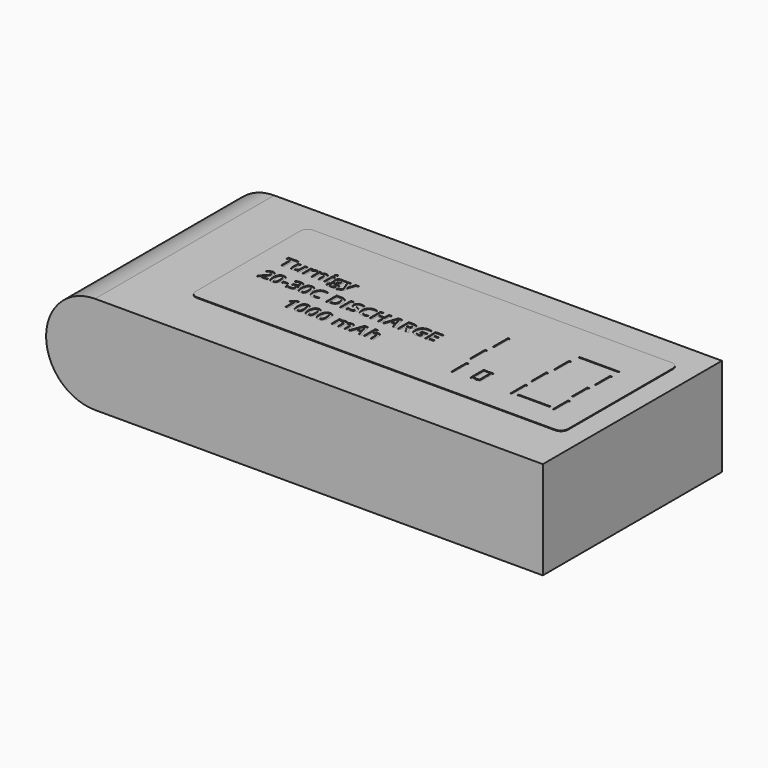
from build123d import *

# Parameters (mm, degrees)
F0_W     = 71
F0_H     = 32
F1_DEPTH = 14
F2_R     = 6.99999
F3_W     = 0.296875
F3_H     = 2.7330729167
F3_W_2   = 0.7282986111
F3_H_2   = 0.3389756944
F3_W_3   = 0.4205729167
F3_H_3   = 1.9830729167
F3_W_4   = 0.4136284722
F3_H_4   = 1.5164930556
F4_DEPTH = 0.1


# Not quite as in the source:
# - a fillet or chamfer is up to 0.001 mm smaller than in the source, because OpenCascade refuses the exact size


with BuildPart() as f1:
    # F0 (on Top) → F1 (new body)
    with BuildSketch(Plane.XY):
        with Locations((-5.0565935671, -0.0620016182)):
            Rectangle(F0_W, F0_H)
    extrude(amount=F1_DEPTH)

    # F2 (radius 7 in the source; OpenCascade refuses exactly that, so slightly less here)
    f2_edges = [f1.edges().sort_by_distance(p)[0] for p in [
        (-40.556594, -0.062002, 14),
        (-40.556594, -0.062002, 0),
    ]]
    fillet(f2_edges, radius=F2_R)

    # F3 (on face) → F4 (join)
    with BuildSketch(Plane.XY.offset(14)):
        with BuildLine():
            Line((26.4446923286, 11.9373770431), (-24.7810670882, 11.9373770431))
            ThreePointArc((-24.7810670882, 11.9373770431), (-25.4881738694, 11.6444838243), (-25.7810670882, 10.9373770431))
            Line((-25.7810670882, 10.9373770431), (-25.7810670882, -7.8157188147))
            ThreePointArc((-25.7810670882, -7.8157188147), (-25.4881738694, -8.5228255959), (-24.7810670882, -8.8157188147))
            Line((-24.7810670882, -8.8157188147), (26.4446923286, -8.8157188147))
            ThreePointArc((26.4446923286, -8.8157188147), (27.1517991098, -8.5228255959), (27.4446923286, -7.8157188147))
            Line((27.4446923286, -7.8157188147), (27.4446923286, 10.9373770431))
            ThreePointArc((27.4446923286, 10.9373770431), (27.1517991098, 11.6444838243), (26.4446923286, 11.9373770431))
        make_face()
        with BuildLine():
            Line((-15.2074745615, -2.5303943503), (-15.2074745615, -4.5134672669))
            Line((-15.2074745615, -4.5134672669), (-15.6267453948, -4.5134672669))
            Line((-15.6267453948, -4.5134672669), (-15.6267453948, -3.3658978225))
            Line((-15.6267453948, -3.3658978225), (-15.6224051171, -3.1775297669))
            Line((-15.6224051171, -3.1775297669), (-15.6158947004, -2.9713665725))
            add(Edge.make_bspline(
                [(-15.6158947004, -2.9713665725), (-15.7200613671, -3.0755332392), (-15.7608599782, -3.1080853225)],
                knots=[0, 0, 0, 1, 1, 1], degree=2))
            Line((-15.7608599782, -3.1080853225), (-15.9887245615, -3.2912450447))
            Line((-15.9887245615, -3.2912450447), (-16.190981506, -3.0390749058))
            Line((-16.190981506, -3.0390749058), (-15.5520926171, -2.5303943503))
            Line((-15.5520926171, -2.5303943503), (-15.2074745615, -2.5303943503))
        make_face(mode=Mode.SUBTRACT)
        with BuildLine():
            add(Edge.make_bspline(
                [(-13.458559631, -2.7595610169), (-13.2829953948, -3.0199776836), (-13.2829953948, -3.5221478225)],
                knots=[0, 0, 0, 1, 1, 1], degree=2))
            add(Edge.make_bspline(
                [(-13.2829953948, -3.5221478225), (-13.2829953948, -4.0412450447), (-13.4531342837, -4.2910280308)],
                knots=[0, 0, 0, 1, 1, 1], degree=2))
            add(Edge.make_bspline(
                [(-13.4531342837, -4.2910280308), (-13.6232731726, -4.5408110169), (-13.9774398393, -4.5408110169)],
                knots=[0, 0, 0, 1, 1, 1], degree=2))
            add(Edge.make_bspline(
                [(-13.9774398393, -4.5408110169), (-14.3207558115, -4.5408110169), (-14.4950179643, -4.2829985169)],
                knots=[0, 0, 0, 1, 1, 1], degree=2))
            add(Edge.make_bspline(
                [(-14.4950179643, -4.2829985169), (-14.6692801171, -4.0251860169), (-14.6692801171, -3.5221478225)],
                knots=[0, 0, 0, 1, 1, 1], degree=2))
            add(Edge.make_bspline(
                [(-14.6692801171, -3.5221478225), (-14.6692801171, -2.9969742114), (-14.499575256, -2.7480592808)],
                knots=[0, 0, 0, 1, 1, 1], degree=2))
            add(Edge.make_bspline(
                [(-14.499575256, -2.7480592808), (-14.3298703948, -2.4991443503), (-13.9774398393, -2.4991443503)],
                knots=[0, 0, 0, 1, 1, 1], degree=2))
            add(Edge.make_bspline(
                [(-13.9774398393, -2.4991443503), (-13.6341238671, -2.4991443503), (-13.458559631, -2.7595610169)],
                knots=[0, 0, 0, 1, 1, 1], degree=2))
        make_face(mode=Mode.SUBTRACT)
        with BuildLine():
            add(Edge.make_bspline(
                [(-11.8730561587, -2.7595610169), (-11.6974919226, -3.0199776836), (-11.6974919226, -3.5221478225)],
                knots=[0, 0, 0, 1, 1, 1], degree=2))
            add(Edge.make_bspline(
                [(-11.6974919226, -3.5221478225), (-11.6974919226, -4.0412450447), (-11.8676308115, -4.2910280308)],
                knots=[0, 0, 0, 1, 1, 1], degree=2))
            add(Edge.make_bspline(
                [(-11.8676308115, -4.2910280308), (-12.0377697004, -4.5408110169), (-12.3919363671, -4.5408110169)],
                knots=[0, 0, 0, 1, 1, 1], degree=2))
            add(Edge.make_bspline(
                [(-12.3919363671, -4.5408110169), (-12.7352523393, -4.5408110169), (-12.9095144921, -4.2829985169)],
                knots=[0, 0, 0, 1, 1, 1], degree=2))
            add(Edge.make_bspline(
                [(-12.9095144921, -4.2829985169), (-13.0837766448, -4.0251860169), (-13.0837766448, -3.5221478225)],
                knots=[0, 0, 0, 1, 1, 1], degree=2))
            add(Edge.make_bspline(
                [(-13.0837766448, -3.5221478225), (-13.0837766448, -2.9969742114), (-12.9140717837, -2.7480592808)],
                knots=[0, 0, 0, 1, 1, 1], degree=2))
            add(Edge.make_bspline(
                [(-12.9140717837, -2.7480592808), (-12.7443669226, -2.4991443503), (-12.3919363671, -2.4991443503)],
                knots=[0, 0, 0, 1, 1, 1], degree=2))
            add(Edge.make_bspline(
                [(-12.3919363671, -2.4991443503), (-12.0486203948, -2.4991443503), (-11.8730561587, -2.7595610169)],
                knots=[0, 0, 0, 1, 1, 1], degree=2))
        make_face(mode=Mode.SUBTRACT)
        with BuildLine():
            add(Edge.make_bspline(
                [(-10.2875526865, -2.7595610169), (-10.1119884504, -3.0199776836), (-10.1119884504, -3.5221478225)],
                knots=[0, 0, 0, 1, 1, 1], degree=2))
            add(Edge.make_bspline(
                [(-10.1119884504, -3.5221478225), (-10.1119884504, -4.0412450447), (-10.2821273393, -4.2910280308)],
                knots=[0, 0, 0, 1, 1, 1], degree=2))
            add(Edge.make_bspline(
                [(-10.2821273393, -4.2910280308), (-10.4522662282, -4.5408110169), (-10.8064328948, -4.5408110169)],
                knots=[0, 0, 0, 1, 1, 1], degree=2))
            add(Edge.make_bspline(
                [(-10.8064328948, -4.5408110169), (-11.1497488671, -4.5408110169), (-11.3240110198, -4.2829985169)],
                knots=[0, 0, 0, 1, 1, 1], degree=2))
            add(Edge.make_bspline(
                [(-11.3240110198, -4.2829985169), (-11.4982731726, -4.0251860169), (-11.4982731726, -3.5221478225)],
                knots=[0, 0, 0, 1, 1, 1], degree=2))
            add(Edge.make_bspline(
                [(-11.4982731726, -3.5221478225), (-11.4982731726, -2.9969742114), (-11.3285683115, -2.7480592808)],
                knots=[0, 0, 0, 1, 1, 1], degree=2))
            add(Edge.make_bspline(
                [(-11.3285683115, -2.7480592808), (-11.1588634504, -2.4991443503), (-10.8064328948, -2.4991443503)],
                knots=[0, 0, 0, 1, 1, 1], degree=2))
            add(Edge.make_bspline(
                [(-10.8064328948, -2.4991443503), (-10.4631169226, -2.4991443503), (-10.2875526865, -2.7595610169)],
                knots=[0, 0, 0, 1, 1, 1], degree=2))
        make_face(mode=Mode.SUBTRACT)
        with BuildLine():
            Line((-7.7165891448, -3.7526165725), (-7.7165891448, -4.5134672669))
            Line((-7.7165891448, -4.5134672669), (-8.1302176171, -4.5134672669))
            Line((-8.1302176171, -4.5134672669), (-8.1302176171, -3.6276165725))
            add(Edge.make_bspline(
                [(-8.1302176171, -3.6276165725), (-8.1302176171, -3.4635540725), (-8.185122131, -3.3815228225)],
                knots=[0, 0, 0, 1, 1, 1], degree=2))
            add(Edge.make_bspline(
                [(-8.185122131, -3.3815228225), (-8.2400266448, -3.2994915725), (-8.3580822004, -3.2994915725)],
                knots=[0, 0, 0, 1, 1, 1], degree=2))
            add(Edge.make_bspline(
                [(-8.3580822004, -3.2994915725), (-8.5169363671, -3.2994915725), (-8.5887679643, -3.4162450447)],
                knots=[0, 0, 0, 1, 1, 1], degree=2))
            add(Edge.make_bspline(
                [(-8.5887679643, -3.4162450447), (-8.6605995615, -3.5329985169), (-8.6605995615, -3.7999256003)],
                knots=[0, 0, 0, 1, 1, 1], degree=2))
            Line((-8.6605995615, -3.7999256003), (-8.6605995615, -4.5134672669))
            Line((-8.6605995615, -4.5134672669), (-9.0742280337, -4.5134672669))
            Line((-9.0742280337, -4.5134672669), (-9.0742280337, -2.9969742114))
            Line((-9.0742280337, -2.9969742114), (-8.7582558115, -2.9969742114))
            Line((-8.7582558115, -2.9969742114), (-8.702700256, -3.1909846281))
            Line((-8.702700256, -3.1909846281), (-8.6796967837, -3.1909846281))
            add(Edge.make_bspline(
                [(-8.6796967837, -3.1909846281), (-8.6184988671, -3.0863839336), (-8.5032644921, -3.0275731697)],
                knots=[0, 0, 0, 1, 1, 1], degree=2))
            add(Edge.make_bspline(
                [(-8.5032644921, -3.0275731697), (-8.3880301171, -2.9687624058), (-8.2387245615, -2.9687624058)],
                knots=[0, 0, 0, 1, 1, 1], degree=2))
            add(Edge.make_bspline(
                [(-8.2387245615, -2.9687624058), (-7.8984467837, -2.9687624058), (-7.7773530337, -3.1909846281)],
                knots=[0, 0, 0, 1, 1, 1], degree=2))
            Line((-7.7773530337, -3.1909846281), (-7.7408947004, -3.1909846281))
            add(Edge.make_bspline(
                [(-7.7408947004, -3.1909846281), (-7.6796967837, -3.0850818503), (-7.5612072004, -3.0269221281)],
                knots=[0, 0, 0, 1, 1, 1], degree=2))
            add(Edge.make_bspline(
                [(-7.5612072004, -3.0269221281), (-7.4427176171, -2.9687624058), (-7.2934120615, -2.9687624058)],
                knots=[0, 0, 0, 1, 1, 1], degree=2))
            add(Edge.make_bspline(
                [(-7.2934120615, -2.9687624058), (-7.0355995615, -2.9687624058), (-6.9034381032, -3.1009238642)],
                knots=[0, 0, 0, 1, 1, 1], degree=2))
            add(Edge.make_bspline(
                [(-6.9034381032, -3.1009238642), (-6.7712766448, -3.2330853225), (-6.7712766448, -3.5247519892)],
                knots=[0, 0, 0, 1, 1, 1], degree=2))
            Line((-6.7712766448, -3.5247519892), (-6.7712766448, -4.5134672669))
            Line((-6.7712766448, -4.5134672669), (-7.1862072004, -4.5134672669))
            Line((-7.1862072004, -4.5134672669), (-7.1862072004, -3.6276165725))
            add(Edge.make_bspline(
                [(-7.1862072004, -3.6276165725), (-7.1862072004, -3.4635540725), (-7.2411117143, -3.3815228225)],
                knots=[0, 0, 0, 1, 1, 1], degree=2))
            add(Edge.make_bspline(
                [(-7.2411117143, -3.3815228225), (-7.2960162282, -3.2994915725), (-7.4140717837, -3.2994915725)],
                knots=[0, 0, 0, 1, 1, 1], degree=2))
            add(Edge.make_bspline(
                [(-7.4140717837, -3.2994915725), (-7.565981506, -3.2994915725), (-7.6412853254, -3.4079985169)],
                knots=[0, 0, 0, 1, 1, 1], degree=2))
            add(Edge.make_bspline(
                [(-7.6412853254, -3.4079985169), (-7.7165891448, -3.5165054614), (-7.7165891448, -3.7526165725)],
                knots=[0, 0, 0, 1, 1, 1], degree=2))
        make_face(mode=Mode.SUBTRACT)
        Polygon((-4.6471447004, -4.5134672669), (-5.1002697004, -4.5134672669), (-5.2439328948, -4.0412450447), (-5.9670231726, -4.0412450447), (-6.1106863671, -4.5134672669), (-6.5638113671, -4.5134672669), (-5.8637245615, -2.5221478225), (-5.3498356726, -2.5221478225), align=None, mode=Mode.SUBTRACT)
        with BuildLine():
            Line((-3.0303912282, -3.5247519892), (-3.0303912282, -4.5134672669))
            Line((-3.0303912282, -4.5134672669), (-3.4440197004, -4.5134672669))
            Line((-3.4440197004, -4.5134672669), (-3.4440197004, -3.6276165725))
            add(Edge.make_bspline(
                [(-3.4440197004, -3.6276165725), (-3.4440197004, -3.2994915725), (-3.6883773393, -3.2994915725)],
                knots=[0, 0, 0, 1, 1, 1], degree=2))
            add(Edge.make_bspline(
                [(-3.6883773393, -3.2994915725), (-3.8619884504, -3.2994915725), (-3.9392453948, -3.4175471281)],
                knots=[0, 0, 0, 1, 1, 1], degree=2))
            add(Edge.make_bspline(
                [(-3.9392453948, -3.4175471281), (-4.0165023393, -3.5356026836), (-4.0165023393, -3.7999256003)],
                knots=[0, 0, 0, 1, 1, 1], degree=2))
            Line((-4.0165023393, -3.7999256003), (-4.0165023393, -4.5134672669))
            Line((-4.0165023393, -4.5134672669), (-4.4301308115, -4.5134672669))
            Line((-4.4301308115, -4.5134672669), (-4.4301308115, -2.4027901836))
            Line((-4.4301308115, -2.4027901836), (-4.0165023393, -2.4027901836))
            Line((-4.0165023393, -2.4027901836), (-4.0165023393, -2.8329117114))
            add(Edge.make_bspline(
                [(-4.0165023393, -2.8329117114), (-4.0165023393, -2.8832589336), (-4.0260509504, -3.0690228225)],
                knots=[0, 0, 0, 1, 1, 1], degree=2))
            Line((-4.0260509504, -3.0690228225), (-4.0355995615, -3.1909846281))
            Line((-4.0355995615, -3.1909846281), (-4.0138981726, -3.1909846281))
            add(Edge.make_bspline(
                [(-4.0138981726, -3.1909846281), (-3.8754433115, -2.9687624058), (-3.5742280337, -2.9687624058)],
                knots=[0, 0, 0, 1, 1, 1], degree=2))
            add(Edge.make_bspline(
                [(-3.5742280337, -2.9687624058), (-3.3068669226, -2.9687624058), (-3.1686290754, -3.1124256003)],
                knots=[0, 0, 0, 1, 1, 1], degree=2))
            add(Edge.make_bspline(
                [(-3.1686290754, -3.1124256003), (-3.0303912282, -3.2560887947), (-3.0303912282, -3.5247519892)],
                knots=[0, 0, 0, 1, 1, 1], degree=2))
        make_face(mode=Mode.SUBTRACT)
        with Locations((8.7708240496, -3.7775731697)):
            Rectangle(F3_W, F3_H, mode=Mode.SUBTRACT)
        Polygon((11.8289837718, -4.6666790725), (11.8289837718, -4.9531374058), (11.1727337718, -4.9531374058), (11.1727337718, -2.5303943503), (11.8289837718, -2.5303943503), (11.8289837718, -2.8168526836), (11.5251643274, -2.8168526836), (11.5251643274, -4.6666790725), align=None, mode=Mode.SUBTRACT)
        Polygon((11.9674386329, -4.9531374058), (11.9674386329, -4.6666790725), (12.269955994, -4.6666790725), (12.269955994, -2.8168526836), (11.9674386329, -2.8168526836), (11.9674386329, -2.5303943503), (12.6241226607, -2.5303943503), (12.6241226607, -4.9531374058), align=None, mode=Mode.SUBTRACT)
        Polygon((20.2352337718, -4.9531374058), (19.1045914107, -4.9531374058), (19.0933066885, -4.9531374058), (17.9513796052, -4.9531374058), (17.9513796052, -4.7630332392), (19.0933066885, -4.7630332392), (19.1045914107, -4.7630332392), (20.2352337718, -4.7630332392), (20.246518494, -4.7630332392), (21.3771608552, -4.7630332392), (21.3884455774, -4.7630332392), (22.5303726607, -4.7630332392), (22.5303726607, -4.9531374058), (21.3884455774, -4.9531374058), (21.3771608552, -4.9531374058), (20.246518494, -4.9531374058), align=None, mode=Mode.SUBTRACT)
        with Locations((17.1926990496, -3.7775731697)):
            Rectangle(F3_W, F3_H, mode=Mode.SUBTRACT)
        with Locations((23.2903552996, -3.7775731697)):
            Rectangle(F3_W, F3_H, mode=Mode.SUBTRACT)
        with BuildLine():
            Line((-21.3537419226, -0.3828249058), (-21.3537419226, -0.7356894892))
            Line((-21.3537419226, -0.7356894892), (-22.7400266448, -0.7356894892))
            Line((-22.7400266448, -0.7356894892), (-22.7400266448, -0.4440228225))
            Line((-22.7400266448, -0.4440228225), (-22.2421967837, 0.0590153719))
            add(Edge.make_bspline(
                [(-22.2421967837, 0.0590153719), (-22.0208426171, 0.2855778719), (-21.9531342837, 0.3730344692)],
                knots=[0, 0, 0, 1, 1, 1], degree=2))
            add(Edge.make_bspline(
                [(-21.9531342837, 0.3730344692), (-21.8854259504, 0.4604910664), (-21.8554780337, 0.5351438442)],
                knots=[0, 0, 0, 1, 1, 1], degree=2))
            add(Edge.make_bspline(
                [(-21.8554780337, 0.5351438442), (-21.8255301171, 0.6097966219), (-21.8255301171, 0.6896577331)],
                knots=[0, 0, 0, 1, 1, 1], degree=2))
            add(Edge.make_bspline(
                [(-21.8255301171, 0.6896577331), (-21.8255301171, 0.8090153719), (-21.8915023393, 0.8673921081)],
                knots=[0, 0, 0, 1, 1, 1], degree=2))
            add(Edge.make_bspline(
                [(-21.8915023393, 0.8673921081), (-21.9574745615, 0.9257688442), (-22.0672835893, 0.9257688442)],
                knots=[0, 0, 0, 1, 1, 1], degree=2))
            add(Edge.make_bspline(
                [(-22.0672835893, 0.9257688442), (-22.1823009504, 0.9257688442), (-22.2908078948, 0.8728174553)],
                knots=[0, 0, 0, 1, 1, 1], degree=2))
            add(Edge.make_bspline(
                [(-22.2908078948, 0.8728174553), (-22.3993148393, 0.8198660664), (-22.5173703948, 0.7222098164)],
                knots=[0, 0, 0, 1, 1, 1], degree=2))
            Line((-22.5173703948, 0.7222098164), (-22.7452349782, 0.9921750942))
            add(Edge.make_bspline(
                [(-22.7452349782, 0.9921750942), (-22.5989676171, 1.1171750942), (-22.5026134504, 1.1686073858)],
                knots=[0, 0, 0, 1, 1, 1], degree=2))
            add(Edge.make_bspline(
                [(-22.5026134504, 1.1686073858), (-22.4062592837, 1.2200396775), (-22.2923269921, 1.2478174553)],
                knots=[0, 0, 0, 1, 1, 1], degree=2))
            add(Edge.make_bspline(
                [(-22.2923269921, 1.2478174553), (-22.1783947004, 1.2755952331), (-22.0373356726, 1.2755952331)],
                knots=[0, 0, 0, 1, 1, 1], degree=2))
            add(Edge.make_bspline(
                [(-22.0373356726, 1.2755952331), (-21.8515717837, 1.2755952331), (-21.7092106726, 1.2078868997)],
                knots=[0, 0, 0, 1, 1, 1], degree=2))
            add(Edge.make_bspline(
                [(-21.7092106726, 1.2078868997), (-21.5668495615, 1.1401785664), (-21.4880735198, 1.0179997469)],
                knots=[0, 0, 0, 1, 1, 1], degree=2))
            add(Edge.make_bspline(
                [(-21.4880735198, 1.0179997469), (-21.4092974782, 0.8958209275), (-21.4092974782, 0.7387028719)],
                knots=[0, 0, 0, 1, 1, 1], degree=2))
            add(Edge.make_bspline(
                [(-21.4092974782, 0.7387028719), (-21.4092974782, 0.6015500942), (-21.4574745615, 0.4815414136)],
                knots=[0, 0, 0, 1, 1, 1], degree=2))
            add(Edge.make_bspline(
                [(-21.4574745615, 0.4815414136), (-21.5056516448, 0.3615327331), (-21.6067801171, 0.2354476636)],
                knots=[0, 0, 0, 1, 1, 1], degree=2))
            add(Edge.make_bspline(
                [(-21.6067801171, 0.2354476636), (-21.7079085893, 0.1093625942), (-21.9626828948, -0.1241443503)],
                knots=[0, 0, 0, 1, 1, 1], degree=2))
            Line((-21.9626828948, -0.1241443503), (-22.2178912282, -0.3641617114))
            Line((-22.2178912282, -0.3641617114), (-22.2178912282, -0.3828249058))
            Line((-22.2178912282, -0.3828249058), (-21.3537419226, -0.3828249058))
        make_face(mode=Mode.SUBTRACT)
        with BuildLine():
            add(Edge.make_bspline(
                [(-19.954653381, 1.0182167608), (-19.7790891448, 0.7578000942), (-19.7790891448, 0.2556299553)],
                knots=[0, 0, 0, 1, 1, 1], degree=2))
            add(Edge.make_bspline(
                [(-19.7790891448, 0.2556299553), (-19.7790891448, -0.2634672669), (-19.9492280337, -0.5132502531)],
                knots=[0, 0, 0, 1, 1, 1], degree=2))
            add(Edge.make_bspline(
                [(-19.9492280337, -0.5132502531), (-20.1193669226, -0.7630332392), (-20.4735335893, -0.7630332392)],
                knots=[0, 0, 0, 1, 1, 1], degree=2))
            add(Edge.make_bspline(
                [(-20.4735335893, -0.7630332392), (-20.8168495615, -0.7630332392), (-20.9911117143, -0.5052207392)],
                knots=[0, 0, 0, 1, 1, 1], degree=2))
            add(Edge.make_bspline(
                [(-20.9911117143, -0.5052207392), (-21.1653738671, -0.2474082392), (-21.1653738671, 0.2556299553)],
                knots=[0, 0, 0, 1, 1, 1], degree=2))
            add(Edge.make_bspline(
                [(-21.1653738671, 0.2556299553), (-21.1653738671, 0.7808035664), (-20.995669006, 1.0297184969)],
                knots=[0, 0, 0, 1, 1, 1], degree=2))
            add(Edge.make_bspline(
                [(-20.995669006, 1.0297184969), (-20.8259641448, 1.2786334275), (-20.4735335893, 1.2786334275)],
                knots=[0, 0, 0, 1, 1, 1], degree=2))
            add(Edge.make_bspline(
                [(-20.4735335893, 1.2786334275), (-20.1302176171, 1.2786334275), (-19.954653381, 1.0182167608)],
                knots=[0, 0, 0, 1, 1, 1], degree=2))
        make_face(mode=Mode.SUBTRACT)
        with Locations((-19.2330822004, 0.0088851636)):
            Rectangle(F3_W_2, F3_H_2, mode=Mode.SUBTRACT)
        with BuildLine():
            add(Edge.make_bspline(
                [(-17.5447141448, 1.1508122469), (-17.3663287282, 1.0260292608), (-17.3663287282, 0.8038070386)],
                knots=[0, 0, 0, 1, 1, 1], degree=2))
            add(Edge.make_bspline(
                [(-17.3663287282, 0.8038070386), (-17.3663287282, 0.6180431497), (-17.4789589365, 0.4878348164)],
                knots=[0, 0, 0, 1, 1, 1], degree=2))
            add(Edge.make_bspline(
                [(-17.4789589365, 0.4878348164), (-17.5915891448, 0.3576264831), (-17.7951481726, 0.3085813442)],
                knots=[0, 0, 0, 1, 1, 1], degree=2))
            Line((-17.7951481726, 0.3085813442), (-17.7951481726, 0.3007688442))
            add(Edge.make_bspline(
                [(-17.7951481726, 0.3007688442), (-17.5546967837, 0.2708209275), (-17.4314328948, 0.1547184969)],
                knots=[0, 0, 0, 1, 1, 1], degree=2))
            add(Edge.make_bspline(
                [(-17.4314328948, 0.1547184969), (-17.308169006, 0.0386160664), (-17.308169006, -0.1579985169)],
                knots=[0, 0, 0, 1, 1, 1], degree=2))
            add(Edge.make_bspline(
                [(-17.308169006, -0.1579985169), (-17.308169006, -0.4440228225), (-17.5156342837, -0.6035280308)],
                knots=[0, 0, 0, 1, 1, 1], degree=2))
            add(Edge.make_bspline(
                [(-17.5156342837, -0.6035280308), (-17.7230995615, -0.7630332392), (-18.1080822004, -0.7630332392)],
                knots=[0, 0, 0, 1, 1, 1], degree=2))
            add(Edge.make_bspline(
                [(-18.1080822004, -0.7630332392), (-18.4309988671, -0.7630332392), (-18.6805648393, -0.6558283781)],
                knots=[0, 0, 0, 1, 1, 1], degree=2))
            Line((-18.6805648393, -0.6558283781), (-18.6805648393, -0.2990575447))
            add(Edge.make_bspline(
                [(-18.6805648393, -0.2990575447), (-18.5655474782, -0.3572172669), (-18.4270926171, -0.3938926142)],
                knots=[0, 0, 0, 1, 1, 1], degree=2))
            add(Edge.make_bspline(
                [(-18.4270926171, -0.3938926142), (-18.288637756, -0.4305679614), (-18.1532210893, -0.4305679614)],
                knots=[0, 0, 0, 1, 1, 1], degree=2))
            add(Edge.make_bspline(
                [(-18.1532210893, -0.4305679614), (-17.9453217837, -0.4305679614), (-17.8463634504, -0.3600384475)],
                knots=[0, 0, 0, 1, 1, 1], degree=2))
            add(Edge.make_bspline(
                [(-17.8463634504, -0.3600384475), (-17.7474051171, -0.2895089336), (-17.7474051171, -0.1332589336)],
                knots=[0, 0, 0, 1, 1, 1], degree=2))
            add(Edge.make_bspline(
                [(-17.7474051171, -0.1332589336), (-17.7474051171, 0.0060639831), (-17.8613374087, 0.0644407192)],
                knots=[0, 0, 0, 1, 1, 1], degree=2))
            add(Edge.make_bspline(
                [(-17.8613374087, 0.0644407192), (-17.9752697004, 0.1228174553), (-18.2248356726, 0.1228174553)],
                knots=[0, 0, 0, 1, 1, 1], degree=2))
            Line((-18.2248356726, 0.1228174553), (-18.3754433115, 0.1228174553))
            Line((-18.3754433115, 0.1228174553), (-18.3754433115, 0.4444320386))
            Line((-18.3754433115, 0.4444320386), (-18.222231506, 0.4444320386))
            add(Edge.make_bspline(
                [(-18.222231506, 0.4444320386), (-17.991762756, 0.4444320386), (-17.8852089365, 0.5047618997)],
                knots=[0, 0, 0, 1, 1, 1], degree=2))
            add(Edge.make_bspline(
                [(-17.8852089365, 0.5047618997), (-17.7786551171, 0.5650917608), (-17.7786551171, 0.7113591219)],
                knots=[0, 0, 0, 1, 1, 1], degree=2))
            add(Edge.make_bspline(
                [(-17.7786551171, 0.7113591219), (-17.7786551171, 0.9366195386), (-18.0607731726, 0.9366195386)],
                knots=[0, 0, 0, 1, 1, 1], degree=2))
            add(Edge.make_bspline(
                [(-18.0607731726, 0.9366195386), (-18.1584294226, 0.9366195386), (-18.2595578948, 0.9040674553)],
                knots=[0, 0, 0, 1, 1, 1], degree=2))
            add(Edge.make_bspline(
                [(-18.2595578948, 0.9040674553), (-18.3606863671, 0.8715153719), (-18.483950256, 0.7916542608)],
                knots=[0, 0, 0, 1, 1, 1], degree=2))
            Line((-18.483950256, 0.7916542608), (-18.6779606726, 1.0802827331))
            add(Edge.make_bspline(
                [(-18.6779606726, 1.0802827331), (-18.4066933115, 1.2755952331), (-18.030825256, 1.2755952331)],
                knots=[0, 0, 0, 1, 1, 1], degree=2))
            add(Edge.make_bspline(
                [(-18.030825256, 1.2755952331), (-17.7230995615, 1.2755952331), (-17.5447141448, 1.1508122469)],
                knots=[0, 0, 0, 1, 1, 1], degree=2))
        make_face(mode=Mode.SUBTRACT)
        with BuildLine():
            Line((-19.6341238671, 3.0420882886), (-19.9513981726, 3.0420882886))
            Line((-19.9513981726, 3.0420882886), (-20.0069537282, 3.2360987053))
            Line((-20.0069537282, 3.2360987053), (-20.0286551171, 3.2360987053))
            add(Edge.make_bspline(
                [(-20.0286551171, 3.2360987053), (-20.0950613671, 3.1301959275), (-20.2172401865, 3.0724702331)],
                knots=[0, 0, 0, 1, 1, 1], degree=2))
            add(Edge.make_bspline(
                [(-20.2172401865, 3.0724702331), (-20.339419006, 3.0147445386), (-20.4952349782, 3.0147445386)],
                knots=[0, 0, 0, 1, 1, 1], degree=2))
            add(Edge.make_bspline(
                [(-20.4952349782, 3.0147445386), (-20.7625960893, 3.0147445386), (-20.8982297698, 3.1579737053)],
                knots=[0, 0, 0, 1, 1, 1], degree=2))
            add(Edge.make_bspline(
                [(-20.8982297698, 3.1579737053), (-21.0338634504, 3.3012028719), (-21.0338634504, 3.5698660664)],
                knots=[0, 0, 0, 1, 1, 1], degree=2))
            Line((-21.0338634504, 3.5698660664), (-21.0338634504, 4.5585813442))
            Line((-21.0338634504, 4.5585813442), (-20.6202349782, 4.5585813442))
            Line((-20.6202349782, 4.5585813442), (-20.6202349782, 3.6727306497))
            add(Edge.make_bspline(
                [(-20.6202349782, 3.6727306497), (-20.6202349782, 3.5086681497), (-20.5618582421, 3.4266368997)],
                knots=[0, 0, 0, 1, 1, 1], degree=2))
            add(Edge.make_bspline(
                [(-20.5618582421, 3.4266368997), (-20.503481506, 3.3446056497), (-20.3758773393, 3.3446056497)],
                knots=[0, 0, 0, 1, 1, 1], degree=2))
            add(Edge.make_bspline(
                [(-20.3758773393, 3.3446056497), (-20.2022662282, 3.3446056497), (-20.1250092837, 3.4604910664)],
                knots=[0, 0, 0, 1, 1, 1], degree=2))
            add(Edge.make_bspline(
                [(-20.1250092837, 3.4604910664), (-20.0477523393, 3.5763764831), (-20.0477523393, 3.8450396775)],
                knots=[0, 0, 0, 1, 1, 1], degree=2))
            Line((-20.0477523393, 3.8450396775), (-20.0477523393, 4.5585813442))
            Line((-20.0477523393, 4.5585813442), (-19.6341238671, 4.5585813442))
            Line((-19.6341238671, 4.5585813442), (-19.6341238671, 3.0420882886))
        make_face(mode=Mode.SUBTRACT)
        with BuildLine():
            add(Edge.make_bspline(
                [(-18.614809631, 4.5088851636), (-18.4948009504, 4.5867931497), (-18.3537419226, 4.5867931497)],
                knots=[0, 0, 0, 1, 1, 1], degree=2))
            add(Edge.make_bspline(
                [(-18.3537419226, 4.5867931497), (-18.2695405337, 4.5867931497), (-18.2139849782, 4.5746403719)],
                knots=[0, 0, 0, 1, 1, 1], degree=2))
            Line((-18.2139849782, 4.5746403719), (-18.2452349782, 4.1870535664))
            add(Edge.make_bspline(
                [(-18.2452349782, 4.1870535664), (-18.2955822004, 4.2005084275), (-18.3671967837, 4.2005084275)],
                knots=[0, 0, 0, 1, 1, 1], degree=2))
            add(Edge.make_bspline(
                [(-18.3671967837, 4.2005084275), (-18.5651134504, 4.2005084275), (-18.6757905337, 4.0987289136)],
                knots=[0, 0, 0, 1, 1, 1], degree=2))
            add(Edge.make_bspline(
                [(-18.6757905337, 4.0987289136), (-18.7864676171, 3.9969493997), (-18.7864676171, 3.8137896775)],
                knots=[0, 0, 0, 1, 1, 1], degree=2))
            Line((-18.7864676171, 3.8137896775), (-18.7864676171, 3.0420882886))
            Line((-18.7864676171, 3.0420882886), (-19.2000960893, 3.0420882886))
            Line((-19.2000960893, 3.0420882886), (-19.2000960893, 4.5585813442))
            Line((-19.2000960893, 4.5585813442), (-18.8867280337, 4.5585813442))
            Line((-18.8867280337, 4.5585813442), (-18.8255301171, 4.3033730108))
            Line((-18.8255301171, 4.3033730108), (-18.8055648393, 4.3033730108))
            add(Edge.make_bspline(
                [(-18.8055648393, 4.3033730108), (-18.7348183115, 4.4309771775), (-18.614809631, 4.5088851636)],
                knots=[0, 0, 0, 1, 1, 1], degree=2))
        make_face(mode=Mode.SUBTRACT)
        Polygon((-21.8363808115, 4.6753348164), (-21.8363808115, 3.0420882886), (-22.2569537282, 3.0420882886), (-22.2569537282, 4.6753348164), (-22.7955822004, 4.6753348164), (-22.7955822004, 5.0251612053), (-21.2981863671, 5.0251612053), (-21.2981863671, 4.6753348164), align=None, mode=Mode.SUBTRACT)
        with BuildLine():
            add(Edge.make_bspline(
                [(-15.8899832421, 1.0182167608), (-15.714419006, 0.7578000942), (-15.714419006, 0.2556299553)],
                knots=[0, 0, 0, 1, 1, 1], degree=2))
            add(Edge.make_bspline(
                [(-15.714419006, 0.2556299553), (-15.714419006, -0.2634672669), (-15.8845578948, -0.5132502531)],
                knots=[0, 0, 0, 1, 1, 1], degree=2))
            add(Edge.make_bspline(
                [(-15.8845578948, -0.5132502531), (-16.0546967837, -0.7630332392), (-16.4088634504, -0.7630332392)],
                knots=[0, 0, 0, 1, 1, 1], degree=2))
            add(Edge.make_bspline(
                [(-16.4088634504, -0.7630332392), (-16.7521794226, -0.7630332392), (-16.9264415754, -0.5052207392)],
                knots=[0, 0, 0, 1, 1, 1], degree=2))
            add(Edge.make_bspline(
                [(-16.9264415754, -0.5052207392), (-17.1007037282, -0.2474082392), (-17.1007037282, 0.2556299553)],
                knots=[0, 0, 0, 1, 1, 1], degree=2))
            add(Edge.make_bspline(
                [(-17.1007037282, 0.2556299553), (-17.1007037282, 0.7808035664), (-16.9309988671, 1.0297184969)],
                knots=[0, 0, 0, 1, 1, 1], degree=2))
            add(Edge.make_bspline(
                [(-16.9309988671, 1.0297184969), (-16.761294006, 1.2786334275), (-16.4088634504, 1.2786334275)],
                knots=[0, 0, 0, 1, 1, 1], degree=2))
            add(Edge.make_bspline(
                [(-16.4088634504, 1.2786334275), (-16.0655474782, 1.2786334275), (-15.8899832421, 1.0182167608)],
                knots=[0, 0, 0, 1, 1, 1], degree=2))
        make_face(mode=Mode.SUBTRACT)
        with BuildLine():
            add(Edge.make_bspline(
                [(-14.3025266448, 0.8864893303), (-14.4149398393, 0.9257688442), (-14.5234467837, 0.9257688442)],
                knots=[0, 0, 0, 1, 1, 1], degree=2))
            add(Edge.make_bspline(
                [(-14.5234467837, 0.9257688442), (-14.7608599782, 0.9257688442), (-14.8910683115, 0.7473834275)],
                knots=[0, 0, 0, 1, 1, 1], degree=2))
            add(Edge.make_bspline(
                [(-14.8910683115, 0.7473834275), (-15.0212766448, 0.5689980108), (-15.0212766448, 0.2504216219)],
                knots=[0, 0, 0, 1, 1, 1], degree=2))
            add(Edge.make_bspline(
                [(-15.0212766448, 0.2504216219), (-15.0212766448, -0.4127728225), (-14.5234467837, -0.4127728225)],
                knots=[0, 0, 0, 1, 1, 1], degree=2))
            add(Edge.make_bspline(
                [(-14.5234467837, -0.4127728225), (-14.3146794226, -0.4127728225), (-14.0178044226, -0.3086061558)],
                knots=[0, 0, 0, 1, 1, 1], degree=2))
            Line((-14.0178044226, -0.3086061558), (-14.0178044226, -0.6610367114))
            add(Edge.make_bspline(
                [(-14.0178044226, -0.6610367114), (-14.2617280337, -0.7630332392), (-14.5629433115, -0.7630332392)],
                knots=[0, 0, 0, 1, 1, 1], degree=2))
            add(Edge.make_bspline(
                [(-14.5629433115, -0.7630332392), (-14.995669006, -0.7630332392), (-15.2248356726, -0.5004464336)],
                knots=[0, 0, 0, 1, 1, 1], degree=2))
            add(Edge.make_bspline(
                [(-15.2248356726, -0.5004464336), (-15.4540023393, -0.2378596281), (-15.4540023393, 0.2530257886)],
                knots=[0, 0, 0, 1, 1, 1], degree=2))
            add(Edge.make_bspline(
                [(-15.4540023393, 0.2530257886), (-15.4540023393, 0.5624875942), (-15.341372131, 0.7951264831)],
                knots=[0, 0, 0, 1, 1, 1], degree=2))
            add(Edge.make_bspline(
                [(-15.341372131, 0.7951264831), (-15.2287419226, 1.0277653719), (-15.0178044226, 1.1516803025)],
                knots=[0, 0, 0, 1, 1, 1], degree=2))
            add(Edge.make_bspline(
                [(-15.0178044226, 1.1516803025), (-14.8068669226, 1.2755952331), (-14.5234467837, 1.2755952331)],
                knots=[0, 0, 0, 1, 1, 1], degree=2))
            add(Edge.make_bspline(
                [(-14.5234467837, 1.2755952331), (-14.2348183115, 1.2755952331), (-13.9431516448, 1.1362723164)],
                knots=[0, 0, 0, 1, 1, 1], degree=2))
            Line((-13.9431516448, 1.1362723164), (-14.0785683115, 0.7942584275))
            add(Edge.make_bspline(
                [(-14.0785683115, 0.7942584275), (-14.1901134504, 0.8472098164), (-14.3025266448, 0.8864893303)],
                knots=[0, 0, 0, 1, 1, 1], degree=2))
        make_face(mode=Mode.SUBTRACT)
        with BuildLine():
            add(Edge.make_bspline(
                [(-11.4974051171, 0.9910900247), (-11.2287419226, 0.7347966219), (-11.2287419226, 0.2747271775)],
                knots=[0, 0, 0, 1, 1, 1], degree=2))
            add(Edge.make_bspline(
                [(-11.2287419226, 0.2747271775), (-11.2287419226, -0.2148561558), (-11.5076047698, -0.4752728225)],
                knots=[0, 0, 0, 1, 1, 1], degree=2))
            add(Edge.make_bspline(
                [(-11.5076047698, -0.4752728225), (-11.7864676171, -0.7356894892), (-12.3125092837, -0.7356894892)],
                knots=[0, 0, 0, 1, 1, 1], degree=2))
            Line((-12.3125092837, -0.7356894892), (-12.8741412282, -0.7356894892))
            Line((-12.8741412282, -0.7356894892), (-12.8741412282, 1.2473834275))
            Line((-12.8741412282, 1.2473834275), (-12.2517453948, 1.2473834275))
            add(Edge.make_bspline(
                [(-12.2517453948, 1.2473834275), (-11.7660683115, 1.2473834275), (-11.4974051171, 0.9910900247)],
                knots=[0, 0, 0, 1, 1, 1], degree=2))
        make_face(mode=Mode.SUBTRACT)
        with Locations((-10.6074311587, 0.2558469692)):
            Rectangle(F3_W_3, F3_H_3, mode=Mode.SUBTRACT)
        with BuildLine():
            Line((-16.5390717837, 4.0308035664), (-16.5390717837, 3.0420882886))
            Line((-16.5390717837, 3.0420882886), (-16.952700256, 3.0420882886))
            Line((-16.952700256, 3.0420882886), (-16.952700256, 3.9279389831))
            add(Edge.make_bspline(
                [(-16.952700256, 3.9279389831), (-16.952700256, 4.0920014831), (-17.0110769921, 4.1740327331)],
                knots=[0, 0, 0, 1, 1, 1], degree=2))
            add(Edge.make_bspline(
                [(-17.0110769921, 4.1740327331), (-17.0694537282, 4.2560639831), (-17.1970578948, 4.2560639831)],
                knots=[0, 0, 0, 1, 1, 1], degree=2))
            add(Edge.make_bspline(
                [(-17.1970578948, 4.2560639831), (-17.370669006, 4.2560639831), (-17.4479259504, 4.1401785664)],
                knots=[0, 0, 0, 1, 1, 1], degree=2))
            add(Edge.make_bspline(
                [(-17.4479259504, 4.1401785664), (-17.5251828948, 4.0242931497), (-17.5251828948, 3.7556299553)],
                knots=[0, 0, 0, 1, 1, 1], degree=2))
            Line((-17.5251828948, 3.7556299553), (-17.5251828948, 3.0420882886))
            Line((-17.5251828948, 3.0420882886), (-17.9388113671, 3.0420882886))
            Line((-17.9388113671, 3.0420882886), (-17.9388113671, 4.5585813442))
            Line((-17.9388113671, 4.5585813442), (-17.6228391448, 4.5585813442))
            Line((-17.6228391448, 4.5585813442), (-17.5672835893, 4.3645709275))
            Line((-17.5672835893, 4.3645709275), (-17.5442801171, 4.3645709275))
            add(Edge.make_bspline(
                [(-17.5442801171, 4.3645709275), (-17.4748356726, 4.4743799553), (-17.3535249087, 4.5305865525)],
                knots=[0, 0, 0, 1, 1, 1], degree=2))
            add(Edge.make_bspline(
                [(-17.3535249087, 4.5305865525), (-17.2322141448, 4.5867931497), (-17.077700256, 4.5867931497)],
                knots=[0, 0, 0, 1, 1, 1], degree=2))
            add(Edge.make_bspline(
                [(-17.077700256, 4.5867931497), (-16.8129433115, 4.5867931497), (-16.6760075476, 4.4437809969)],
                knots=[0, 0, 0, 1, 1, 1], degree=2))
            add(Edge.make_bspline(
                [(-16.6760075476, 4.4437809969), (-16.5390717837, 4.3007688442), (-16.5390717837, 4.0308035664)],
                knots=[0, 0, 0, 1, 1, 1], degree=2))
        make_face(mode=Mode.SUBTRACT)
        with Locations((-15.9064762976, 3.8003348164)):
            Rectangle(F3_W_4, F3_H_4, mode=Mode.SUBTRACT)
        with BuildLine():
            Line((-14.4748356726, 4.5585813442), (-13.9457558115, 4.5585813442))
            Line((-13.9457558115, 4.5585813442), (-13.9457558115, 4.3480778719))
            Line((-13.9457558115, 4.3480778719), (-14.183169006, 4.2873139831))
            add(Edge.make_bspline(
                [(-14.183169006, 4.2873139831), (-14.1180648393, 4.1853174553), (-14.1180648393, 4.0594493997)],
                knots=[0, 0, 0, 1, 1, 1], degree=2))
            add(Edge.make_bspline(
                [(-14.1180648393, 4.0594493997), (-14.1180648393, 3.8150917608), (-14.2884207421, 3.6788070386)],
                knots=[0, 0, 0, 1, 1, 1], degree=2))
            add(Edge.make_bspline(
                [(-14.2884207421, 3.6788070386), (-14.4587766448, 3.5425223164), (-14.7608599782, 3.5425223164)],
                knots=[0, 0, 0, 1, 1, 1], degree=2))
            Line((-14.7608599782, 3.5425223164), (-14.835512756, 3.5468625942))
            Line((-14.835512756, 3.5468625942), (-14.8967106726, 3.5533730108))
            add(Edge.make_bspline(
                [(-14.8967106726, 3.5533730108), (-14.960512756, 3.5047618997), (-14.960512756, 3.4448660664)],
                knots=[0, 0, 0, 1, 1, 1], degree=2))
            add(Edge.make_bspline(
                [(-14.960512756, 3.4448660664), (-14.960512756, 3.3554563442), (-14.7326481726, 3.3554563442)],
                knots=[0, 0, 0, 1, 1, 1], degree=2))
            Line((-14.7326481726, 3.3554563442), (-14.4748356726, 3.3554563442))
            add(Edge.make_bspline(
                [(-14.4748356726, 3.3554563442), (-14.2252697004, 3.3554563442), (-14.0944103254, 3.2482514831)],
                knots=[0, 0, 0, 1, 1, 1], degree=2))
            add(Edge.make_bspline(
                [(-14.0944103254, 3.2482514831), (-13.9635509504, 3.1410466219), (-13.9635509504, 2.9335813442)],
                knots=[0, 0, 0, 1, 1, 1], degree=2))
            add(Edge.make_bspline(
                [(-13.9635509504, 2.9335813442), (-13.9635509504, 2.6675223164), (-14.1853391448, 2.5210379414)],
                knots=[0, 0, 0, 1, 1, 1], degree=2))
            add(Edge.make_bspline(
                [(-14.1853391448, 2.5210379414), (-14.4071273393, 2.3745535664), (-14.8220578948, 2.3745535664)],
                knots=[0, 0, 0, 1, 1, 1], degree=2))
            add(Edge.make_bspline(
                [(-14.8220578948, 2.3745535664), (-15.1393322004, 2.3745535664), (-15.3068669226, 2.4852306497)],
                knots=[0, 0, 0, 1, 1, 1], degree=2))
            add(Edge.make_bspline(
                [(-15.3068669226, 2.4852306497), (-15.4744016448, 2.5959077331), (-15.4744016448, 2.7951264831)],
                knots=[0, 0, 0, 1, 1, 1], degree=2))
            add(Edge.make_bspline(
                [(-15.4744016448, 2.7951264831), (-15.4744016448, 2.9322792608), (-15.3888981726, 3.0245101636)],
                knots=[0, 0, 0, 1, 1, 1], degree=2))
            add(Edge.make_bspline(
                [(-15.3888981726, 3.0245101636), (-15.3033947004, 3.1167410664), (-15.1380301171, 3.1562375942)],
                knots=[0, 0, 0, 1, 1, 1], degree=2))
            add(Edge.make_bspline(
                [(-15.1380301171, 3.1562375942), (-15.2018322004, 3.1831473164), (-15.2493582421, 3.2447792608)],
                knots=[0, 0, 0, 1, 1, 1], degree=2))
            add(Edge.make_bspline(
                [(-15.2493582421, 3.2447792608), (-15.2968842837, 3.3064112053), (-15.2968842837, 3.3758556497)],
                knots=[0, 0, 0, 1, 1, 1], degree=2))
            add(Edge.make_bspline(
                [(-15.2968842837, 3.3758556497), (-15.2968842837, 3.4626612053), (-15.2467540754, 3.5201698858)],
                knots=[0, 0, 0, 1, 1, 1], degree=2))
            add(Edge.make_bspline(
                [(-15.2467540754, 3.5201698858), (-15.1966238671, 3.5776785664), (-15.1015717837, 3.6336681497)],
                knots=[0, 0, 0, 1, 1, 1], degree=2))
            add(Edge.make_bspline(
                [(-15.1015717837, 3.6336681497), (-15.2209294226, 3.6848834275), (-15.2908078948, 3.7988157192)],
                knots=[0, 0, 0, 1, 1, 1], degree=2))
            add(Edge.make_bspline(
                [(-15.2908078948, 3.7988157192), (-15.3606863671, 3.9127480108), (-15.3606863671, 4.0676959275)],
                knots=[0, 0, 0, 1, 1, 1], degree=2))
            add(Edge.make_bspline(
                [(-15.3606863671, 4.0676959275), (-15.3606863671, 4.3155257886), (-15.1992280337, 4.4511594692)],
                knots=[0, 0, 0, 1, 1, 1], degree=2))
            add(Edge.make_bspline(
                [(-15.1992280337, 4.4511594692), (-15.0377697004, 4.5867931497), (-14.737856506, 4.5867931497)],
                knots=[0, 0, 0, 1, 1, 1], degree=2))
            add(Edge.make_bspline(
                [(-14.737856506, 4.5867931497), (-14.6740544226, 4.5867931497), (-14.5865978254, 4.5752914136)],
                knots=[0, 0, 0, 1, 1, 1], degree=2))
            add(Edge.make_bspline(
                [(-14.5865978254, 4.5752914136), (-14.4991412282, 4.5637896775), (-14.4748356726, 4.5585813442)],
                knots=[0, 0, 0, 1, 1, 1], degree=2))
        make_face(mode=Mode.SUBTRACT)
        with BuildLine():
            Line((-13.3107731726, 3.0529389831), (-13.9132037282, 4.5585813442))
            Line((-13.9132037282, 4.5585813442), (-13.4600787282, 4.5585813442))
            Line((-13.4600787282, 4.5585813442), (-13.1740544226, 3.7052827331))
            add(Edge.make_bspline(
                [(-13.1740544226, 3.7052827331), (-13.1371620615, 3.5941716219), (-13.1237072004, 3.4422618997)],
                knots=[0, 0, 0, 1, 1, 1], degree=2))
            Line((-13.1237072004, 3.4422618997), (-13.1154606726, 3.4422618997))
            add(Edge.make_bspline(
                [(-13.1154606726, 3.4422618997), (-13.1007037282, 3.5820188442), (-13.0573009504, 3.7052827331)],
                knots=[0, 0, 0, 1, 1, 1], degree=2))
            Line((-13.0573009504, 3.7052827331), (-12.7764849782, 4.5585813442))
            Line((-12.7764849782, 4.5585813442), (-12.3329085893, 4.5585813442))
            Line((-12.3329085893, 4.5585813442), (-12.9744016448, 2.8480778719))
            add(Edge.make_bspline(
                [(-12.9744016448, 2.8480778719), (-13.0629433115, 2.6106646775), (-13.2263547698, 2.4926091219)],
                knots=[0, 0, 0, 1, 1, 1], degree=2))
            add(Edge.make_bspline(
                [(-13.2263547698, 2.4926091219), (-13.3897662282, 2.3745535664), (-13.6080822004, 2.3745535664)],
                knots=[0, 0, 0, 1, 1, 1], degree=2))
            add(Edge.make_bspline(
                [(-13.6080822004, 2.3745535664), (-13.7152870615, 2.3745535664), (-13.8181516448, 2.3979910664)],
                knots=[0, 0, 0, 1, 1, 1], degree=2))
            Line((-13.8181516448, 2.3979910664), (-13.8181516448, 2.7261160664))
            add(Edge.make_bspline(
                [(-13.8181516448, 2.7261160664), (-13.7434988671, 2.7083209275), (-13.6553912282, 2.7083209275)],
                knots=[0, 0, 0, 1, 1, 1], degree=2))
            add(Edge.make_bspline(
                [(-13.6553912282, 2.7083209275), (-13.5455822004, 2.7083209275), (-13.4635509504, 2.7755952331)],
                knots=[0, 0, 0, 1, 1, 1], degree=2))
            add(Edge.make_bspline(
                [(-13.4635509504, 2.7755952331), (-13.3815197004, 2.8428695386), (-13.335512756, 2.9782862053)],
                knots=[0, 0, 0, 1, 1, 1], degree=2))
            Line((-13.335512756, 2.9782862053), (-13.3107731726, 3.0529389831))
        make_face(mode=Mode.SUBTRACT)
        with BuildLine():
            add(Edge.make_bspline(
                [(-8.8305214365, 0.1425657192), (-8.7274398393, 0.0091021775), (-8.7274398393, -0.1849082392)],
                knots=[0, 0, 0, 1, 1, 1], degree=2))
            add(Edge.make_bspline(
                [(-8.7274398393, -0.1849082392), (-8.7274398393, -0.4535714336), (-8.9207992143, -0.6083023364)],
                knots=[0, 0, 0, 1, 1, 1], degree=2))
            add(Edge.make_bspline(
                [(-8.9207992143, -0.6083023364), (-9.1141585893, -0.7630332392), (-9.4583426171, -0.7630332392)],
                knots=[0, 0, 0, 1, 1, 1], degree=2))
            add(Edge.make_bspline(
                [(-9.4583426171, -0.7630332392), (-9.7760509504, -0.7630332392), (-10.0199745615, -0.6432415725)],
                knots=[0, 0, 0, 1, 1, 1], degree=2))
            Line((-10.0199745615, -0.6432415725), (-10.0199745615, -0.2526165725))
            add(Edge.make_bspline(
                [(-10.0199745615, -0.2526165725), (-9.8194537282, -0.3424603225), (-9.6803478254, -0.3789186558)],
                knots=[0, 0, 0, 1, 1, 1], degree=2))
            add(Edge.make_bspline(
                [(-9.6803478254, -0.3789186558), (-9.5412419226, -0.4153769892), (-9.4257905337, -0.4153769892)],
                knots=[0, 0, 0, 1, 1, 1], degree=2))
            add(Edge.make_bspline(
                [(-9.4257905337, -0.4153769892), (-9.2877697004, -0.4153769892), (-9.2137679643, -0.3626426142)],
                knots=[0, 0, 0, 1, 1, 1], degree=2))
            add(Edge.make_bspline(
                [(-9.2137679643, -0.3626426142), (-9.1397662282, -0.3099082392), (-9.1397662282, -0.2053075447)],
                knots=[0, 0, 0, 1, 1, 1], degree=2))
            add(Edge.make_bspline(
                [(-9.1397662282, -0.2053075447), (-9.1397662282, -0.1471478225), (-9.1723183115, -0.1015749058)],
                knots=[0, 0, 0, 1, 1, 1], degree=2))
            add(Edge.make_bspline(
                [(-9.1723183115, -0.1015749058), (-9.2048703948, -0.0560019892), (-9.2680214365, -0.0141183086)],
                knots=[0, 0, 0, 1, 1, 1], degree=2))
            add(Edge.make_bspline(
                [(-9.2680214365, -0.0141183086), (-9.3311724782, 0.0277653719), (-9.5251828948, 0.1202132886)],
                knots=[0, 0, 0, 1, 1, 1], degree=2))
            add(Edge.make_bspline(
                [(-9.5251828948, 0.1202132886), (-9.706606506, 0.2057167608), (-9.7975353254, 0.2842757886)],
                knots=[0, 0, 0, 1, 1, 1], degree=2))
            add(Edge.make_bspline(
                [(-9.7975353254, 0.2842757886), (-9.8884641448, 0.3628348164), (-9.9427176171, 0.4674355108)],
                knots=[0, 0, 0, 1, 1, 1], degree=2))
            add(Edge.make_bspline(
                [(-9.9427176171, 0.4674355108), (-9.9969710893, 0.5720362053), (-9.9969710893, 0.7113591219)],
                knots=[0, 0, 0, 1, 1, 1], degree=2))
            add(Edge.make_bspline(
                [(-9.9969710893, 0.7113591219), (-9.9969710893, 0.9748139831), (-9.8185856726, 1.1252046081)],
                knots=[0, 0, 0, 1, 1, 1], degree=2))
            add(Edge.make_bspline(
                [(-9.8185856726, 1.1252046081), (-9.640200256, 1.2755952331), (-9.3255301171, 1.2755952331)],
                knots=[0, 0, 0, 1, 1, 1], degree=2))
            add(Edge.make_bspline(
                [(-9.3255301171, 1.2755952331), (-9.1710162282, 1.2755952331), (-9.0306082421, 1.2391368997)],
                knots=[0, 0, 0, 1, 1, 1], degree=2))
            add(Edge.make_bspline(
                [(-9.0306082421, 1.2391368997), (-8.890200256, 1.2026785664), (-8.7369884504, 1.1362723164)],
                knots=[0, 0, 0, 1, 1, 1], degree=2))
            Line((-8.7369884504, 1.1362723164), (-8.8724051171, 0.8090153719))
            add(Edge.make_bspline(
                [(-8.8724051171, 0.8090153719), (-9.0312592837, 0.8741195386), (-9.1349919226, 0.8999441914)],
                knots=[0, 0, 0, 1, 1, 1], degree=2))
            add(Edge.make_bspline(
                [(-9.1349919226, 0.8999441914), (-9.2387245615, 0.9257688442), (-9.3389849782, 0.9257688442)],
                knots=[0, 0, 0, 1, 1, 1], degree=2))
            add(Edge.make_bspline(
                [(-9.3389849782, 0.9257688442), (-9.4583426171, 0.9257688442), (-9.5221447004, 0.8702132886)],
                knots=[0, 0, 0, 1, 1, 1], degree=2))
            add(Edge.make_bspline(
                [(-9.5221447004, 0.8702132886), (-9.5859467837, 0.8146577331), (-9.5859467837, 0.7252480108)],
                knots=[0, 0, 0, 1, 1, 1], degree=2))
            add(Edge.make_bspline(
                [(-9.5859467837, 0.7252480108), (-9.5859467837, 0.6696924553), (-9.560122131, 0.6282428025)],
                knots=[0, 0, 0, 1, 1, 1], degree=2))
            add(Edge.make_bspline(
                [(-9.560122131, 0.6282428025), (-9.5342974782, 0.5867931497), (-9.478090881, 0.5481646775)],
                knots=[0, 0, 0, 1, 1, 1], degree=2))
            add(Edge.make_bspline(
                [(-9.478090881, 0.5481646775), (-9.4218842837, 0.5095362053), (-9.2118148393, 0.4092757886)],
                knots=[0, 0, 0, 1, 1, 1], degree=2))
            add(Edge.make_bspline(
                [(-9.2118148393, 0.4092757886), (-8.9336030337, 0.2760292608), (-8.8305214365, 0.1425657192)],
                knots=[0, 0, 0, 1, 1, 1], degree=2))
        make_face(mode=Mode.SUBTRACT)
        with BuildLine():
            add(Edge.make_bspline(
                [(-7.3046967837, 0.8864893303), (-7.4171099782, 0.9257688442), (-7.5256169226, 0.9257688442)],
                knots=[0, 0, 0, 1, 1, 1], degree=2))
            add(Edge.make_bspline(
                [(-7.5256169226, 0.9257688442), (-7.7630301171, 0.9257688442), (-7.8932384504, 0.7473834275)],
                knots=[0, 0, 0, 1, 1, 1], degree=2))
            add(Edge.make_bspline(
                [(-7.8932384504, 0.7473834275), (-8.0234467837, 0.5689980108), (-8.0234467837, 0.2504216219)],
                knots=[0, 0, 0, 1, 1, 1], degree=2))
            add(Edge.make_bspline(
                [(-8.0234467837, 0.2504216219), (-8.0234467837, -0.4127728225), (-7.5256169226, -0.4127728225)],
                knots=[0, 0, 0, 1, 1, 1], degree=2))
            add(Edge.make_bspline(
                [(-7.5256169226, -0.4127728225), (-7.3168495615, -0.4127728225), (-7.0199745615, -0.3086061558)],
                knots=[0, 0, 0, 1, 1, 1], degree=2))
            Line((-7.0199745615, -0.3086061558), (-7.0199745615, -0.6610367114))
            add(Edge.make_bspline(
                [(-7.0199745615, -0.6610367114), (-7.2638981726, -0.7630332392), (-7.5651134504, -0.7630332392)],
                knots=[0, 0, 0, 1, 1, 1], degree=2))
            add(Edge.make_bspline(
                [(-7.5651134504, -0.7630332392), (-7.9978391448, -0.7630332392), (-8.2270058115, -0.5004464336)],
                knots=[0, 0, 0, 1, 1, 1], degree=2))
            add(Edge.make_bspline(
                [(-8.2270058115, -0.5004464336), (-8.4561724782, -0.2378596281), (-8.4561724782, 0.2530257886)],
                knots=[0, 0, 0, 1, 1, 1], degree=2))
            add(Edge.make_bspline(
                [(-8.4561724782, 0.2530257886), (-8.4561724782, 0.5624875942), (-8.3435422698, 0.7951264831)],
                knots=[0, 0, 0, 1, 1, 1], degree=2))
            add(Edge.make_bspline(
                [(-8.3435422698, 0.7951264831), (-8.2309120615, 1.0277653719), (-8.0199745615, 1.1516803025)],
                knots=[0, 0, 0, 1, 1, 1], degree=2))
            add(Edge.make_bspline(
                [(-8.0199745615, 1.1516803025), (-7.8090370615, 1.2755952331), (-7.5256169226, 1.2755952331)],
                knots=[0, 0, 0, 1, 1, 1], degree=2))
            add(Edge.make_bspline(
                [(-7.5256169226, 1.2755952331), (-7.2369884504, 1.2755952331), (-6.9453217837, 1.1362723164)],
                knots=[0, 0, 0, 1, 1, 1], degree=2))
            Line((-6.9453217837, 1.1362723164), (-7.0807384504, 0.7942584275))
            add(Edge.make_bspline(
                [(-7.0807384504, 0.7942584275), (-7.1922835893, 0.8472098164), (-7.3046967837, 0.8864893303)],
                knots=[0, 0, 0, 1, 1, 1], degree=2))
        make_face(mode=Mode.SUBTRACT)
        Polygon((-4.9730995615, 1.2473834275), (-4.9730995615, -0.7356894892), (-5.3923703948, -0.7356894892), (-5.3923703948, 0.1202132886), (-6.1775266448, 0.1202132886), (-6.1775266448, -0.7356894892), (-6.5980995615, -0.7356894892), (-6.5980995615, 1.2473834275), (-6.1775266448, 1.2473834275), (-6.1775266448, 0.4700396775), (-5.3923703948, 0.4700396775), (-5.3923703948, 1.2473834275), align=None, mode=Mode.SUBTRACT)
        Polygon((-2.8055648393, -0.7356894892), (-3.2586898393, -0.7356894892), (-3.4023530337, -0.2634672669), (-4.1254433115, -0.2634672669), (-4.269106506, -0.7356894892), (-4.722231506, -0.7356894892), (-4.0221447004, 1.2556299553), (-3.5082558115, 1.2556299553), align=None, mode=Mode.SUBTRACT)
        with BuildLine():
            Line((-1.9119016448, 0.0251612053), (-2.1354259504, 0.0251612053))
            Line((-2.1354259504, 0.0251612053), (-2.1354259504, -0.7356894892))
            Line((-2.1354259504, -0.7356894892), (-2.5559988671, -0.7356894892))
            Line((-2.5559988671, -0.7356894892), (-2.5559988671, 1.2473834275))
            Line((-2.5559988671, 1.2473834275), (-1.9783078948, 1.2473834275))
            add(Edge.make_bspline(
                [(-1.9783078948, 1.2473834275), (-1.573794006, 1.2473834275), (-1.3800006032, 1.1002480108)],
                knots=[0, 0, 0, 1, 1, 1], degree=2))
            add(Edge.make_bspline(
                [(-1.3800006032, 1.1002480108), (-1.1862072004, 0.9531125942), (-1.1862072004, 0.6531993997)],
                knots=[0, 0, 0, 1, 1, 1], degree=2))
            add(Edge.make_bspline(
                [(-1.1862072004, 0.6531993997), (-1.1862072004, 0.4782862053), (-1.2823443532, 0.3420014831)],
                knots=[0, 0, 0, 1, 1, 1], degree=2))
            add(Edge.make_bspline(
                [(-1.2823443532, 0.3420014831), (-1.378481506, 0.2057167608), (-1.5551308115, 0.1284598164)],
                knots=[0, 0, 0, 1, 1, 1], degree=2))
            add(Edge.make_bspline(
                [(-1.5551308115, 0.1284598164), (-1.1072141448, -0.5403769892), (-0.9717974782, -0.7356894892)],
                knots=[0, 0, 0, 1, 1, 1], degree=2))
            Line((-0.9717974782, -0.7356894892), (-1.4383773393, -0.7356894892))
            Line((-1.4383773393, -0.7356894892), (-1.9119016448, 0.0251612053))
        make_face(mode=Mode.SUBTRACT)
        with BuildLine():
            add(Edge.make_bspline(
                [(-15.905825256, 4.7469493997), (-16.1310856726, 4.7469493997), (-16.1310856726, 4.9505084275)],
                knots=[0, 0, 0, 1, 1, 1], degree=2))
            add(Edge.make_bspline(
                [(-16.1310856726, 4.9505084275), (-16.1310856726, 5.1527653719), (-15.905825256, 5.1527653719)],
                knots=[0, 0, 0, 1, 1, 1], degree=2))
            add(Edge.make_bspline(
                [(-15.905825256, 5.1527653719), (-15.6805648393, 5.1527653719), (-15.6805648393, 4.9505084275)],
                knots=[0, 0, 0, 1, 1, 1], degree=2))
            add(Edge.make_bspline(
                [(-15.6805648393, 4.9505084275), (-15.6805648393, 4.8541542608), (-15.7367714365, 4.8005518303)],
                knots=[0, 0, 0, 1, 1, 1], degree=2))
            add(Edge.make_bspline(
                [(-15.7367714365, 4.8005518303), (-15.7929780337, 4.7469493997), (-15.905825256, 4.7469493997)],
                knots=[0, 0, 0, 1, 1, 1], degree=2))
        make_face(mode=Mode.SUBTRACT)
        with BuildLine():
            Line((0.0303726607, 0.0277653719), (0.0303726607, 0.3780257886))
            Line((0.0303726607, 0.3780257886), (0.8172650218, 0.3780257886))
            Line((0.8172650218, 0.3780257886), (0.8172650218, -0.6501860169))
            add(Edge.make_bspline(
                [(0.8172650218, -0.6501860169), (0.6258587718, -0.7126860169), (0.4570219663, -0.7378596281)],
                knots=[0, 0, 0, 1, 1, 1], degree=2))
            add(Edge.make_bspline(
                [(0.4570219663, -0.7378596281), (0.2881851607, -0.7630332392), (0.1119698829, -0.7630332392)],
                knots=[0, 0, 0, 1, 1, 1], degree=2))
            add(Edge.make_bspline(
                [(0.1119698829, -0.7630332392), (-0.3368148393, -0.7630332392), (-0.5735769921, -0.4991443503)],
                knots=[0, 0, 0, 1, 1, 1], degree=2))
            add(Edge.make_bspline(
                [(-0.5735769921, -0.4991443503), (-0.8103391448, -0.2352554614), (-0.8103391448, 0.2586681497)],
                knots=[0, 0, 0, 1, 1, 1], degree=2))
            add(Edge.make_bspline(
                [(-0.8103391448, 0.2586681497), (-0.8103391448, 0.7387028719), (-0.5355995615, 1.0071490525)],
                knots=[0, 0, 0, 1, 1, 1], degree=2))
            add(Edge.make_bspline(
                [(-0.5355995615, 1.0071490525), (-0.2608599782, 1.2755952331), (0.2256851607, 1.2755952331)],
                knots=[0, 0, 0, 1, 1, 1], degree=2))
            add(Edge.make_bspline(
                [(0.2256851607, 1.2755952331), (0.5312407163, 1.2755952331), (0.8146608552, 1.1536334275)],
                knots=[0, 0, 0, 1, 1, 1], degree=2))
            Line((0.8146608552, 1.1536334275), (0.6749039107, 0.8172618997))
            add(Edge.make_bspline(
                [(0.6749039107, 0.8172618997), (0.4578900218, 0.9257688442), (0.223080994, 0.9257688442)],
                knots=[0, 0, 0, 1, 1, 1], degree=2))
            add(Edge.make_bspline(
                [(0.223080994, 0.9257688442), (-0.0494884504, 0.9257688442), (-0.2135509504, 0.7426091219)],
                knots=[0, 0, 0, 1, 1, 1], degree=2))
            add(Edge.make_bspline(
                [(-0.2135509504, 0.7426091219), (-0.3776134504, 0.5594493997), (-0.3776134504, 0.2504216219)],
                knots=[0, 0, 0, 1, 1, 1], degree=2))
            add(Edge.make_bspline(
                [(-0.3776134504, 0.2504216219), (-0.3776134504, -0.0724950447), (-0.2454519921, -0.2426339336)],
                knots=[0, 0, 0, 1, 1, 1], degree=2))
            add(Edge.make_bspline(
                [(-0.2454519921, -0.2426339336), (-0.1132905337, -0.4127728225), (0.1388796052, -0.4127728225)],
                knots=[0, 0, 0, 1, 1, 1], degree=2))
            add(Edge.make_bspline(
                [(0.1388796052, -0.4127728225), (0.2708240496, -0.4127728225), (0.4062407163, -0.3858631003)],
                knots=[0, 0, 0, 1, 1, 1], degree=2))
            Line((0.4062407163, -0.3858631003), (0.4062407163, 0.0277653719))
            Line((0.4062407163, 0.0277653719), (0.0303726607, 0.0277653719))
        make_face(mode=Mode.SUBTRACT)
        Polygon((2.4309802996, -0.3884672669), (2.4309802996, -0.7356894892), (1.2890532163, -0.7356894892), (1.2890532163, 1.2473834275), (2.4309802996, 1.2473834275), (2.4309802996, 0.9027653719), (1.7096261329, 0.9027653719), (1.7096261329, 0.4674355108), (2.3810671052, 0.4674355108), (2.3810671052, 0.1228174553), (1.7096261329, 0.1228174553), (1.7096261329, -0.3884672669), align=None, mode=Mode.SUBTRACT)
        with Locations((8.4131851607, 0.0002046081)):
            Rectangle(F3_W, F3_H, mode=Mode.SUBTRACT)
        with Locations((8.6427858552, 3.7779823858)):
            Rectangle(F3_W, F3_H, mode=Mode.SUBTRACT)
        with Locations((17.1610150218, 0.0002046081)):
            Rectangle(F3_W, F3_H, mode=Mode.SUBTRACT)
        with Locations((17.3906157163, 3.7779823858)):
            Rectangle(F3_W, F3_H, mode=Mode.SUBTRACT)
        with Locations((23.0216921052, 0.0002046081)):
            Rectangle(F3_W, F3_H, mode=Mode.SUBTRACT)
        with Locations((23.2512927996, 3.7779823858)):
            Rectangle(F3_W, F3_H, mode=Mode.SUBTRACT)
        Polygon((19.8472129385, 6.3801959275), (18.7165705774, 6.3801959275), (18.7052858552, 6.3801959275), (17.5633587718, 6.3801959275), (17.5633587718, 6.5703000942), (18.7052858552, 6.5703000942), (18.7165705774, 6.5703000942), (19.8472129385, 6.5703000942), (19.8584976607, 6.5703000942), (20.9891400218, 6.5703000942), (21.000424744, 6.5703000942), (22.1310671052, 6.5703000942), (22.1423518274, 6.5703000942), (23.2842789107, 6.5703000942), (23.2842789107, 6.3801959275), (22.1423518274, 6.3801959275), (22.1310671052, 6.3801959275), (21.000424744, 6.3801959275), (20.9891400218, 6.3801959275), (19.8584976607, 6.3801959275), align=None, mode=Mode.SUBTRACT)
        with BuildLine():
            add(Edge.make_bspline(
                [(-12.2734467837, -0.3884672669), (-11.6658078948, -0.3884672669), (-11.6658078948, 0.2638764831)],
                knots=[0, 0, 0, 1, 1, 1], degree=2))
            add(Edge.make_bspline(
                [(-11.6658078948, 0.2638764831), (-11.6658078948, 0.9027653719), (-12.230044006, 0.9027653719)],
                knots=[0, 0, 0, 1, 1, 1], degree=2))
            Line((-12.230044006, 0.9027653719), (-12.4535683115, 0.9027653719))
            Line((-12.4535683115, 0.9027653719), (-12.4535683115, -0.3884672669))
            Line((-12.4535683115, -0.3884672669), (-12.2734467837, -0.3884672669))
        make_face()
        with BuildLine():
            add(Edge.make_bspline(
                [(-20.685122131, 0.7799355108), (-20.7487072004, 0.6206473164), (-20.7487072004, 0.2556299553)],
                knots=[0, 0, 0, 1, 1, 1], degree=2))
            add(Edge.make_bspline(
                [(-20.7487072004, 0.2556299553), (-20.7487072004, -0.1089533781), (-20.6857731726, -0.2669394892)],
                knots=[0, 0, 0, 1, 1, 1], degree=2))
            add(Edge.make_bspline(
                [(-20.6857731726, -0.2669394892), (-20.6228391448, -0.4249256003), (-20.4735335893, -0.4249256003)],
                knots=[0, 0, 0, 1, 1, 1], degree=2))
            add(Edge.make_bspline(
                [(-20.4735335893, -0.4249256003), (-20.3268322004, -0.4249256003), (-20.2617280337, -0.2649863642)],
                knots=[0, 0, 0, 1, 1, 1], degree=2))
            add(Edge.make_bspline(
                [(-20.2617280337, -0.2649863642), (-20.1966238671, -0.1050471281), (-20.1966238671, 0.2556299553)],
                knots=[0, 0, 0, 1, 1, 1], degree=2))
            add(Edge.make_bspline(
                [(-20.1966238671, 0.2556299553), (-20.1966238671, 0.6206473164), (-20.2625960893, 0.7799355108)],
                knots=[0, 0, 0, 1, 1, 1], degree=2))
            add(Edge.make_bspline(
                [(-20.2625960893, 0.7799355108), (-20.3285683115, 0.9392237053), (-20.4735335893, 0.9392237053)],
                knots=[0, 0, 0, 1, 1, 1], degree=2))
            add(Edge.make_bspline(
                [(-20.4735335893, 0.9392237053), (-20.6215370615, 0.9392237053), (-20.685122131, 0.7799355108)],
                knots=[0, 0, 0, 1, 1, 1], degree=2))
        make_face()
        with BuildLine():
            add(Edge.make_bspline(
                [(-16.6204519921, 0.7799355108), (-16.6840370615, 0.6206473164), (-16.6840370615, 0.2556299553)],
                knots=[0, 0, 0, 1, 1, 1], degree=2))
            add(Edge.make_bspline(
                [(-16.6840370615, 0.2556299553), (-16.6840370615, -0.1089533781), (-16.6211030337, -0.2669394892)],
                knots=[0, 0, 0, 1, 1, 1], degree=2))
            add(Edge.make_bspline(
                [(-16.6211030337, -0.2669394892), (-16.558169006, -0.4249256003), (-16.4088634504, -0.4249256003)],
                knots=[0, 0, 0, 1, 1, 1], degree=2))
            add(Edge.make_bspline(
                [(-16.4088634504, -0.4249256003), (-16.2621620615, -0.4249256003), (-16.1970578948, -0.2649863642)],
                knots=[0, 0, 0, 1, 1, 1], degree=2))
            add(Edge.make_bspline(
                [(-16.1970578948, -0.2649863642), (-16.1319537282, -0.1050471281), (-16.1319537282, 0.2556299553)],
                knots=[0, 0, 0, 1, 1, 1], degree=2))
            add(Edge.make_bspline(
                [(-16.1319537282, 0.2556299553), (-16.1319537282, 0.6206473164), (-16.1979259504, 0.7799355108)],
                knots=[0, 0, 0, 1, 1, 1], degree=2))
            add(Edge.make_bspline(
                [(-16.1979259504, 0.7799355108), (-16.2638981726, 0.9392237053), (-16.4088634504, 0.9392237053)],
                knots=[0, 0, 0, 1, 1, 1], degree=2))
            add(Edge.make_bspline(
                [(-16.4088634504, 0.9392237053), (-16.5568669226, 0.9392237053), (-16.6204519921, 0.7799355108)],
                knots=[0, 0, 0, 1, 1, 1], degree=2))
        make_face()
        with BuildLine():
            add(Edge.make_bspline(
                [(-11.0180214365, -2.9978422669), (-11.081606506, -3.1571304614), (-11.081606506, -3.5221478225)],
                knots=[0, 0, 0, 1, 1, 1], degree=2))
            add(Edge.make_bspline(
                [(-11.081606506, -3.5221478225), (-11.081606506, -3.8867311558), (-11.0186724782, -4.0447172669)],
                knots=[0, 0, 0, 1, 1, 1], degree=2))
            add(Edge.make_bspline(
                [(-11.0186724782, -4.0447172669), (-10.9557384504, -4.2027033781), (-10.8064328948, -4.2027033781)],
                knots=[0, 0, 0, 1, 1, 1], degree=2))
            add(Edge.make_bspline(
                [(-10.8064328948, -4.2027033781), (-10.659731506, -4.2027033781), (-10.5946273393, -4.0427641419)],
                knots=[0, 0, 0, 1, 1, 1], degree=2))
            add(Edge.make_bspline(
                [(-10.5946273393, -4.0427641419), (-10.5295231726, -3.8828249058), (-10.5295231726, -3.5221478225)],
                knots=[0, 0, 0, 1, 1, 1], degree=2))
            add(Edge.make_bspline(
                [(-10.5295231726, -3.5221478225), (-10.5295231726, -3.1571304614), (-10.5954953948, -2.9978422669)],
                knots=[0, 0, 0, 1, 1, 1], degree=2))
            add(Edge.make_bspline(
                [(-10.5954953948, -2.9978422669), (-10.6614676171, -2.8385540725), (-10.8064328948, -2.8385540725)],
                knots=[0, 0, 0, 1, 1, 1], degree=2))
            add(Edge.make_bspline(
                [(-10.8064328948, -2.8385540725), (-10.9544363671, -2.8385540725), (-11.0180214365, -2.9978422669)],
                knots=[0, 0, 0, 1, 1, 1], degree=2))
        make_face()
        with BuildLine():
            add(Edge.make_bspline(
                [(-12.6035249087, -2.9978422669), (-12.6671099782, -3.1571304614), (-12.6671099782, -3.5221478225)],
                knots=[0, 0, 0, 1, 1, 1], degree=2))
            add(Edge.make_bspline(
                [(-12.6671099782, -3.5221478225), (-12.6671099782, -3.8867311558), (-12.6041759504, -4.0447172669)],
                knots=[0, 0, 0, 1, 1, 1], degree=2))
            add(Edge.make_bspline(
                [(-12.6041759504, -4.0447172669), (-12.5412419226, -4.2027033781), (-12.3919363671, -4.2027033781)],
                knots=[0, 0, 0, 1, 1, 1], degree=2))
            add(Edge.make_bspline(
                [(-12.3919363671, -4.2027033781), (-12.2452349782, -4.2027033781), (-12.1801308115, -4.0427641419)],
                knots=[0, 0, 0, 1, 1, 1], degree=2))
            add(Edge.make_bspline(
                [(-12.1801308115, -4.0427641419), (-12.1150266448, -3.8828249058), (-12.1150266448, -3.5221478225)],
                knots=[0, 0, 0, 1, 1, 1], degree=2))
            add(Edge.make_bspline(
                [(-12.1150266448, -3.5221478225), (-12.1150266448, -3.1571304614), (-12.1809988671, -2.9978422669)],
                knots=[0, 0, 0, 1, 1, 1], degree=2))
            add(Edge.make_bspline(
                [(-12.1809988671, -2.9978422669), (-12.2469710893, -2.8385540725), (-12.3919363671, -2.8385540725)],
                knots=[0, 0, 0, 1, 1, 1], degree=2))
            add(Edge.make_bspline(
                [(-12.3919363671, -2.8385540725), (-12.5399398393, -2.8385540725), (-12.6035249087, -2.9978422669)],
                knots=[0, 0, 0, 1, 1, 1], degree=2))
        make_face()
        with BuildLine():
            add(Edge.make_bspline(
                [(-14.189028381, -2.9978422669), (-14.2526134504, -3.1571304614), (-14.2526134504, -3.5221478225)],
                knots=[0, 0, 0, 1, 1, 1], degree=2))
            add(Edge.make_bspline(
                [(-14.2526134504, -3.5221478225), (-14.2526134504, -3.8867311558), (-14.1896794226, -4.0447172669)],
                knots=[0, 0, 0, 1, 1, 1], degree=2))
            add(Edge.make_bspline(
                [(-14.1896794226, -4.0447172669), (-14.1267453948, -4.2027033781), (-13.9774398393, -4.2027033781)],
                knots=[0, 0, 0, 1, 1, 1], degree=2))
            add(Edge.make_bspline(
                [(-13.9774398393, -4.2027033781), (-13.8307384504, -4.2027033781), (-13.7656342837, -4.0427641419)],
                knots=[0, 0, 0, 1, 1, 1], degree=2))
            add(Edge.make_bspline(
                [(-13.7656342837, -4.0427641419), (-13.7005301171, -3.8828249058), (-13.7005301171, -3.5221478225)],
                knots=[0, 0, 0, 1, 1, 1], degree=2))
            add(Edge.make_bspline(
                [(-13.7005301171, -3.5221478225), (-13.7005301171, -3.1571304614), (-13.7665023393, -2.9978422669)],
                knots=[0, 0, 0, 1, 1, 1], degree=2))
            add(Edge.make_bspline(
                [(-13.7665023393, -2.9978422669), (-13.8324745615, -2.8385540725), (-13.9774398393, -2.8385540725)],
                knots=[0, 0, 0, 1, 1, 1], degree=2))
            add(Edge.make_bspline(
                [(-13.9774398393, -2.8385540725), (-14.1254433115, -2.8385540725), (-14.189028381, -2.9978422669)],
                knots=[0, 0, 0, 1, 1, 1], degree=2))
        make_face()
        with BuildLine():
            add(Edge.make_bspline(
                [(-15.0397228254, 2.9693886358), (-15.1163287282, 2.9157862053), (-15.1163287282, 2.8276785664)],
                knots=[0, 0, 0, 1, 1, 1], degree=2))
            add(Edge.make_bspline(
                [(-15.1163287282, 2.8276785664), (-15.1163287282, 2.7421750942), (-15.0342974782, 2.6933469692)],
                knots=[0, 0, 0, 1, 1, 1], degree=2))
            add(Edge.make_bspline(
                [(-15.0342974782, 2.6933469692), (-14.9522662282, 2.6445188442), (-14.804262756, 2.6445188442)],
                knots=[0, 0, 0, 1, 1, 1], degree=2))
            add(Edge.make_bspline(
                [(-14.804262756, 2.6445188442), (-14.5820405337, 2.6445188442), (-14.4559554643, 2.7057167608)],
                knots=[0, 0, 0, 1, 1, 1], degree=2))
            add(Edge.make_bspline(
                [(-14.4559554643, 2.7057167608), (-14.3298703948, 2.7669146775), (-14.3298703948, 2.8723834275)],
                knots=[0, 0, 0, 1, 1, 1], degree=2))
            add(Edge.make_bspline(
                [(-14.3298703948, 2.8723834275), (-14.3298703948, 2.9578868997), (-14.4043061587, 2.9904389831)],
                knots=[0, 0, 0, 1, 1, 1], degree=2))
            add(Edge.make_bspline(
                [(-14.4043061587, 2.9904389831), (-14.4787419226, 3.0229910664), (-14.6349919226, 3.0229910664)],
                knots=[0, 0, 0, 1, 1, 1], degree=2))
            Line((-14.6349919226, 3.0229910664), (-14.8494016448, 3.0229910664))
            add(Edge.make_bspline(
                [(-14.8494016448, 3.0229910664), (-14.9631169226, 3.0229910664), (-15.0397228254, 2.9693886358)],
                knots=[0, 0, 0, 1, 1, 1], degree=2))
        make_face()
        with BuildLine():
            Line((-2.1354259504, 0.9027653719), (-2.1354259504, 0.3671750942))
            Line((-2.1354259504, 0.3671750942), (-2.0000092837, 0.3671750942))
            add(Edge.make_bspline(
                [(-2.0000092837, 0.3671750942), (-1.800356506, 0.3671750942), (-1.7055214365, 0.4335813442)],
                knots=[0, 0, 0, 1, 1, 1], degree=2))
            add(Edge.make_bspline(
                [(-1.7055214365, 0.4335813442), (-1.6106863671, 0.4999875942), (-1.6106863671, 0.6423487053)],
                knots=[0, 0, 0, 1, 1, 1], degree=2))
            add(Edge.make_bspline(
                [(-1.6106863671, 0.6423487053), (-1.6106863671, 0.7834077331), (-1.7076915754, 0.8430865525)],
                knots=[0, 0, 0, 1, 1, 1], degree=2))
            add(Edge.make_bspline(
                [(-1.7076915754, 0.8430865525), (-1.8046967837, 0.9027653719), (-2.0078217837, 0.9027653719)],
                knots=[0, 0, 0, 1, 1, 1], degree=2))
            Line((-2.0078217837, 0.9027653719), (-2.1354259504, 0.9027653719))
        make_face()
        with BuildLine():
            Line((-4.0195405337, 0.0889632886), (-3.5030474782, 0.0889632886))
            add(Edge.make_bspline(
                [(-3.5030474782, 0.0889632886), (-3.7022662282, 0.7304563442), (-3.7274398393, 0.8146577331)],
                knots=[0, 0, 0, 1, 1, 1], degree=2))
            add(Edge.make_bspline(
                [(-3.7274398393, 0.8146577331), (-3.7526134504, 0.8988591219), (-3.7634641448, 0.9474702331)],
                knots=[0, 0, 0, 1, 1, 1], degree=2))
            add(Edge.make_bspline(
                [(-3.7634641448, 0.9474702331), (-3.808169006, 0.7738591219), (-4.0195405337, 0.0889632886)],
                knots=[0, 0, 0, 1, 1, 1], degree=2))
        make_face()
        with BuildLine():
            Line((-5.8611203948, -3.6888144892), (-5.3446273393, -3.6888144892))
            add(Edge.make_bspline(
                [(-5.3446273393, -3.6888144892), (-5.5438460893, -3.0473214336), (-5.5690197004, -2.9631200447)],
                knots=[0, 0, 0, 1, 1, 1], degree=2))
            add(Edge.make_bspline(
                [(-5.5690197004, -2.9631200447), (-5.5941933115, -2.8789186558), (-5.605044006, -2.8303075447)],
                knots=[0, 0, 0, 1, 1, 1], degree=2))
            add(Edge.make_bspline(
                [(-5.605044006, -2.8303075447), (-5.6497488671, -3.0039186558), (-5.8611203948, -3.6888144892)],
                knots=[0, 0, 0, 1, 1, 1], degree=2))
        make_face()
        with BuildLine():
            add(Edge.make_bspline(
                [(-14.737856506, 4.3359250942), (-14.9657210893, 4.3359250942), (-14.9657210893, 4.0620535664)],
                knots=[0, 0, 0, 1, 1, 1], degree=2))
            add(Edge.make_bspline(
                [(-14.9657210893, 4.0620535664), (-14.9657210893, 3.9387896775), (-14.9095144921, 3.8667410664)],
                knots=[0, 0, 0, 1, 1, 1], degree=2))
            add(Edge.make_bspline(
                [(-14.9095144921, 3.8667410664), (-14.8533078948, 3.7946924553), (-14.737856506, 3.7946924553)],
                knots=[0, 0, 0, 1, 1, 1], degree=2))
            add(Edge.make_bspline(
                [(-14.737856506, 3.7946924553), (-14.6215370615, 3.7946924553), (-14.5672835893, 3.8667410664)],
                knots=[0, 0, 0, 1, 1, 1], degree=2))
            add(Edge.make_bspline(
                [(-14.5672835893, 3.8667410664), (-14.5130301171, 3.9387896775), (-14.5130301171, 4.0620535664)],
                knots=[0, 0, 0, 1, 1, 1], degree=2))
            add(Edge.make_bspline(
                [(-14.5130301171, 4.0620535664), (-14.5130301171, 4.3359250942), (-14.737856506, 4.3359250942)],
                knots=[0, 0, 0, 1, 1, 1], degree=2))
        make_face()
    extrude(amount=F4_DEPTH)


solid = f1.part
